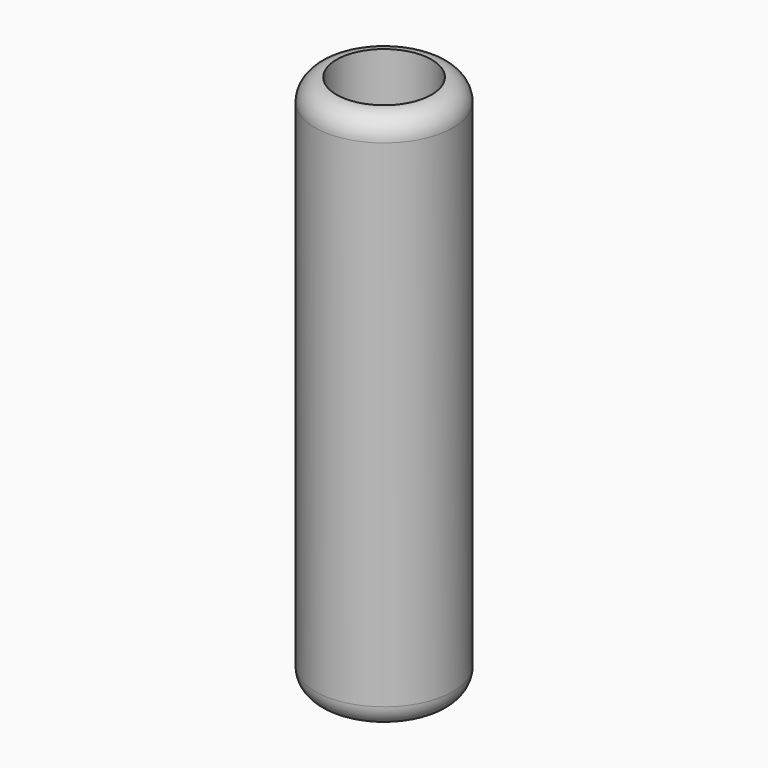
from build123d import *

# Parameters (mm, degrees)
F0_R     = 16
F0_R_2   = 11
F1_DEPTH = 125


# Not quite as in the source:
# - a fillet or chamfer that OpenCascade refuses, or shapes differently, is made with other operations: its cross-section is extruded or revolved along the edge and cut away or added


with BuildPart() as f1:
    # F0 (on Top) → F1 (new body)
    with BuildSketch(Plane.XY):
        Circle(F0_R)
        Circle(F0_R_2, mode=Mode.SUBTRACT)
    extrude(amount=F1_DEPTH)

    # F2: fillet of radius 5.08 on 1 edges, made by hand

    # F2_s1 → F2_t2 (revolve, cut)
    with BuildSketch(Plane.XZ):
        with BuildLine():
            ThreePointArc((16, 119.92), (14.5121024484, 123.5121024484), (10.92, 125))
            Line((10.92, 125), (16, 125))
            Line((16, 125), (16, 119.92))
        make_face()
    revolve(axis=Axis((0, 0, 125), (0, 0, 1)), mode=Mode.SUBTRACT)

    # F3: fillet of radius 5.08 on 1 edges, made by hand

    # F3_s1 → F3_t2 (revolve, cut)
    with BuildSketch(Plane.XZ):
        with BuildLine():
            ThreePointArc((16, 5.08), (14.5121024484, 1.4878975516), (10.92, 0))
            Line((10.92, 0), (16, 0))
            Line((16, 0), (16, 5.08))
        make_face()
    revolve(axis=Axis((0, 0, 0), (0, 0, 1)), mode=Mode.SUBTRACT)


solid = f1.part
